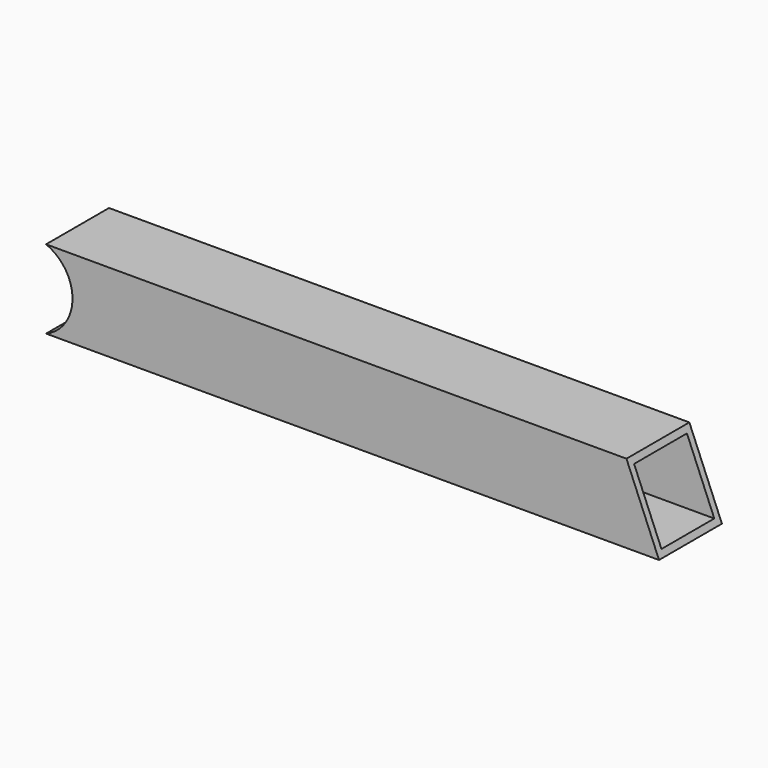
from build123d import *

# Parameters (mm, degrees)
F0_W        = 25
F0_H        = 25
F0_W_2      = 21
F0_H_2      = 21
F1_DEPTH    = 200
F2_T1_DEPTH = 154.6335196453
F3_R        = 13.5
F4_DEPTH    = 25


# Not quite as in the source:
# - a fillet or chamfer that OpenCascade refuses, or shapes differently, is made with other operations: its cross-section is extruded or revolved along the edge and cut away or added


with BuildPart() as f1:
    # F0 (on Right) → F1 (new body)
    with BuildSketch(Plane.YZ):
        Rectangle(F0_W, F0_H)
        Rectangle(F0_W_2, F0_H_2, mode=Mode.SUBTRACT)
    extrude(amount=F1_DEPTH)

    # F2: chamfer of 25 x 10.3553390593 on 1 edges, made by hand

    # F2_s2 → F2_t1 (cut)
    with BuildSketch(Plane.XZ.offset(-77.3167598227)):
        Polygon((189.6446609407, 12.5), (200, -12.5), (200, 12.5), align=None)
    extrude(amount=F2_T1_DEPTH, mode=Mode.SUBTRACT)

    # F3 (on face) → F4 (cut)
    with BuildSketch(Plane.XZ.offset(12.5)):
        Circle(F3_R)
    extrude(amount=-F4_DEPTH, mode=Mode.SUBTRACT)


solid = f1.part
